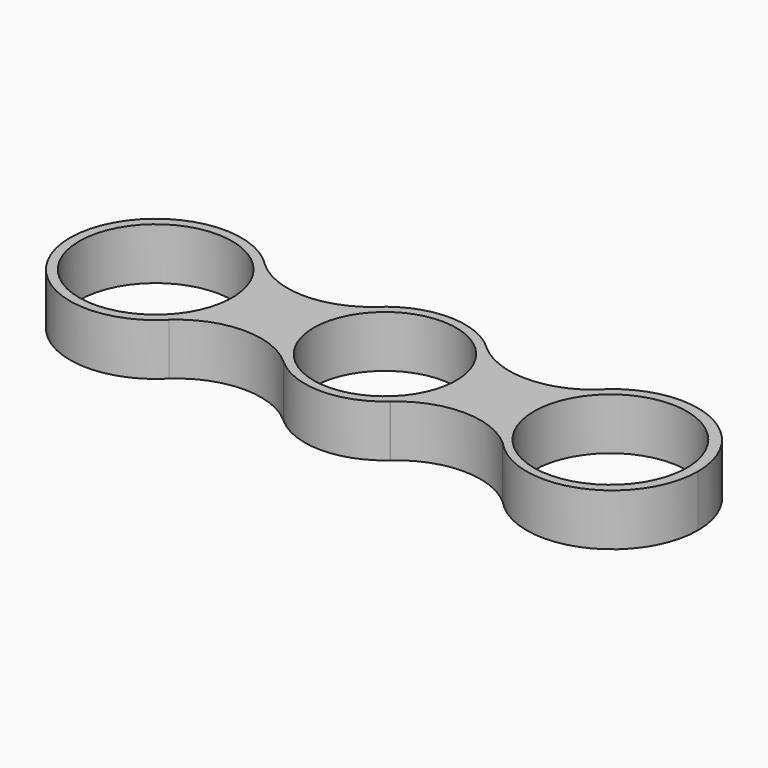
from build123d import *

# Parameters (mm, degrees)
F1_DEPTH = 8
F3_DEPTH = 8
F4_D     = 23.6
F5_D     = 22


# Not quite as in the source:
# - a feature names something its author has since deleted; it is built from what else it names


with BuildPart() as f1:
    # F0 (on Top) → F1 (new body)
    with BuildSketch(Plane.XY):
        with BuildLine():
            ThreePointArc((30.2364596242, 25.5677551031), (18.556965651, 37.3204786398), (6.7314716859, 25.7146705041))
            ThreePointArc((6.7314716859, 25.7146705041), (18.4100473802, 13.8150315665), (30.2364596242, 25.5677551031))
        make_face()
    extrude(amount=F1_DEPTH)

    # F2 (on face) → F3 (join)
    with BuildSketch(Plane.XY.offset(8)):
        with BuildLine():
            ThreePointArc((-42.5114348153, 35.1915450581), (-65.2620832709, 26.0556201481), (-42.5726949965, 16.7685975444))
            ThreePointArc((-42.5726949965, 16.7685975444), (-39.7847972392, 21.021355147), (-38.8073447634, 26.0116364807))
            ThreePointArc((-38.8073447634, 26.0116364807), (-39.7682713179, 30.9611567757), (-42.5114348153, 35.1915450581))
        make_face()
        with BuildLine():
            ThreePointArc((-38.8073447634, 26.0116364807), (-39.7847972392, 21.021355147), (-42.5726949965, 16.7685975444))
            ThreePointArc((-42.5726949965, 16.7685975444), (-33.87370444, 20.218317429), (-25.1016516698, 16.9588551759))
            ThreePointArc((-25.1016516698, 16.9588551759), (-29.0338445102, 25.8480071098), (-25.3315074449, 34.8353238892))
            ThreePointArc((-25.3315074449, 34.8353238892), (-33.9883630197, 31.7873549926), (-42.5114348153, 35.1915450581))
            ThreePointArc((-42.5114348153, 35.1915450581), (-39.7682713179, 30.9611567757), (-38.8073447634, 26.0116364807))
        make_face()
        with BuildLine():
            ThreePointArc((-24.8354704192, 16.7176675443), (-24.9677312973, 16.8391770918), (-25.1016516698, 16.9588551759))
            ThreePointArc((-25.1016516698, 16.9588551759), (-24.9694362403, 16.8372954701), (-24.8354704192, 16.7176675443))
        make_face()
        with BuildLine():
            ThreePointArc((-25.3315074449, 34.8353238892), (-29.0338445102, 25.8480071098), (-25.1016516698, 16.9588551759))
            ThreePointArc((-25.1016516698, 16.9588551759), (-24.9677312973, 16.8391770918), (-24.8354704192, 16.7176675443))
            ThreePointArc((-24.8354704192, 16.7176675443), (-16.6524528686, 13.6328843719), (-8.4735280262, 16.7285025458))
            ThreePointArc((-8.4735280262, 16.7285025458), (-8.4359829057, 16.7620336333), (-8.3983087423, 16.7954196681))
            ThreePointArc((-8.3983087423, 16.7954196681), (-5.3610604956, 20.9632278118), (-4.2864270488, 26.0071017784))
            ThreePointArc((-4.2864270488, 26.0071017784), (-5.2792843636, 30.8636339026), (-8.098530607, 34.9408290832))
            ThreePointArc((-8.098530607, 34.9408290832), (-16.7364042498, 38.381089997), (-25.3315074449, 34.8353238892))
        make_face()
        with BuildLine():
            ThreePointArc((8.8624930635, 34.5276918287), (0.3063045577, 31.6274145181), (-8.098530607, 34.9408290832))
            ThreePointArc((-8.098530607, 34.9408290832), (-5.2792843636, 30.8636339026), (-4.2864270488, 26.0071017784))
            ThreePointArc((-4.2864270488, 26.0071017784), (-5.3610604956, 20.9632278118), (-8.3983087423, 16.7954196681))
            ThreePointArc((-8.3983087423, 16.7954196681), (0.2487240262, 20.0624034029), (8.8910160496, 16.7828993238))
            ThreePointArc((8.8910160496, 16.7828993238), (5.4597887201, 25.6498031441), (8.8624930635, 34.5276918287))
        make_face()
        with BuildLine():
            ThreePointArc((-8.3983087423, 16.7954196681), (-8.4359829057, 16.7620336333), (-8.4735280262, 16.7285025458))
            ThreePointArc((-8.4735280262, 16.7285025458), (-8.4358503291, 16.7618846084), (-8.3983087423, 16.7954196681))
        make_face()
        with BuildLine():
            ThreePointArc((31.9145832669, 25.6710648537), (23.431077599, 38.0185211111), (8.8624930635, 34.5276918287))
            ThreePointArc((8.8624930635, 34.5276918287), (5.4597887201, 25.6498031441), (8.8910160496, 16.7828993238))
            ThreePointArc((8.8910160496, 16.7828993238), (23.4509187507, 13.3312498845), (31.9145832669, 25.6710648537))
        make_face()
    extrude(amount=F3_DEPTH)

    # F4 (through all)
    with Locations(Plane(origin=(0, 0, 0), x_dir=(1, 0, 0), z_dir=(0, 0, -1))):
        with Locations((-52.0347505808, -26.0116364807), (18.4835065156, -25.5677551031)):
            Hole(F4_D / 2)

    # F5 (through all)
    with Locations(Plane(origin=(0, 0, 0), x_dir=(1, 0, 0), z_dir=(0, 0, -1))):
        with Locations((-16.6606471685, -26.0071017784)):
            Hole(F5_D / 2)


solid = f1.part
